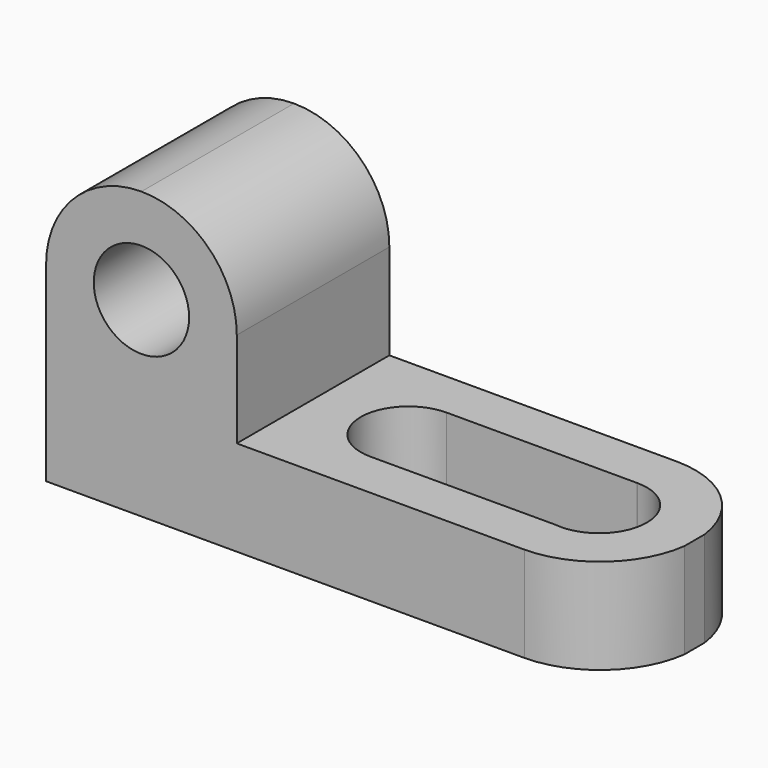
from build123d import *

# Parameters (mm, degrees)
F1_DEPTH = 25.4
F2_R     = 6.35
F3_DEPTH = 25.401
F5_DEPTH = 12.701


with BuildPart() as f1:
    # F0 (on Front) → F1 (new body)
    with BuildSketch(Plane.XZ):
        Polygon((25.4, 38.1), (0, 38.1), (0, 0), (76.2, 0), (76.2, 12.7), (25.4, 12.7), align=None)
    extrude(amount=F1_DEPTH)

    # F2 (on face) → F3 (cut, through all)
    with BuildSketch(Plane.XZ.offset(25.4)):
        with BuildLine():
            ThreePointArc((12.7, 38.1), (21.6802561211, 34.3802561211), (25.4, 25.4))
            Line((25.4, 25.4), (25.4, 38.1))
            Line((25.4, 38.1), (12.7, 38.1))
        make_face()
        with BuildLine():
            ThreePointArc((0, 25.4), (3.7197438789, 34.3802561211), (12.7, 38.1))
            Line((12.7, 38.1), (0, 38.1))
            Line((0, 38.1), (0, 25.4))
        make_face()
        with Locations((12.7, 25.4)):
            Circle(F2_R)
    extrude(amount=-F3_DEPTH, mode=Mode.SUBTRACT)

    # F4 (on face) → F5 (cut, through all)
    with BuildSketch(Plane.XY.offset(12.7)):
        with BuildLine():
            ThreePointArc((62.7121742217, -19.000938862), (57.1631081372, -12.2921991677), (63.526302235, -6.3500544733))
            Line((63.526302235, -6.3500544733), (38.1000136042, -6.35))
            ThreePointArc((38.1000136042, -6.35), (42.5901328704, -8.2098767493), (44.45, -12.7))
            ThreePointArc((44.45, -12.7), (42.5946022143, -17.1856494441), (38.1126611227, -19.0499873776))
            Line((38.1126611227, -19.0499873776), (62.7121742217, -19.000938862))
        make_face()
        with BuildLine():
            ThreePointArc((62.7121742217, -19.000938862), (67.7023687551, -17.4605248498), (69.85, -12.7))
            ThreePointArc((69.85, -12.7), (67.9994176952, -8.2191808334), (63.526302235, -6.3500544733))
            ThreePointArc((63.526302235, -6.3500544733), (57.1631081372, -12.2921991677), (62.7121742217, -19.000938862))
        make_face()
        with BuildLine():
            ThreePointArc((44.45, -12.7), (42.5901328704, -8.2098767493), (38.1000136042, -6.35))
            ThreePointArc((38.1000136042, -6.35), (31.7500031488, -12.7063237624), (38.1126611227, -19.0499873776))
            ThreePointArc((38.1126611227, -19.0499873776), (42.5946022143, -17.1856494441), (44.45, -12.7))
        make_face()
        with BuildLine():
            ThreePointArc((76.2, -14.3920371238), (72.006340741, -22.2314236966), (63.6995432817, -25.4))
            Line((63.6995432817, -25.4), (76.2, -25.4))
            Line((76.2, -25.4), (76.2, -14.3920371238))
        make_face()
        with BuildLine():
            ThreePointArc((63.6995432817, 0), (72.006340741, -3.1685763034), (76.2, -11.0079628762))
            Line((76.2, -11.0079628762), (76.2, 0))
            Line((76.2, 0), (63.6995432817, 0))
        make_face()
    extrude(amount=-F5_DEPTH, mode=Mode.SUBTRACT)


solid = f1.part
